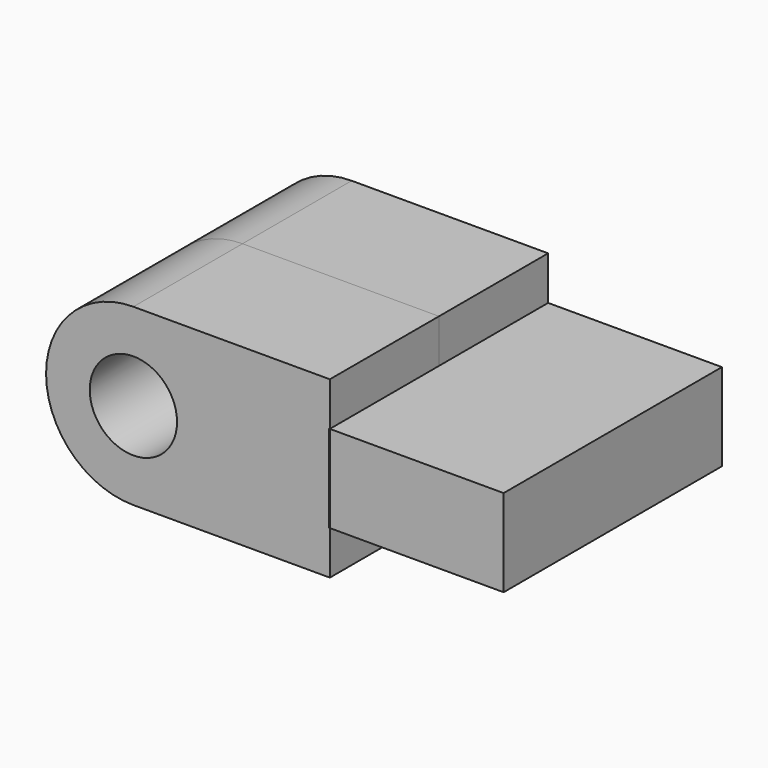
from build123d import *

# Parameters (mm, degrees)
F0_W     = 31.8502481282
F0_H     = 16
F1_DEPTH = 25
F0_R     = 8


with BuildPart() as f1:
    # F0 (on Front) → F1 (new body)
    with BuildSketch(Plane.XZ):
        with Locations((51.9251240641, 0)):
            Rectangle(F0_W, F0_H)
    extrude(amount=F1_DEPTH)

    # F3: F1 across plane


with BuildPart() as f1b:
    # F0 (on Front) → F1, piece 2 (new body)
    with BuildSketch(Plane.XZ):
        with BuildLine():
            Line((36, 16), (0, 16))
            ThreePointArc((0, 16), (-16, 0), (0, -16))
            Line((0, -16), (36, -16))
            Line((36, -16), (36, -8))
            Line((36, -8), (35.8502481282, -8))
            Line((35.8502481282, -8), (35.8502481282, 8))
            Line((35.8502481282, 8), (36, 8))
            Line((36, 8), (36, 16))
        make_face()
        Circle(F0_R, mode=Mode.SUBTRACT)
    extrude(amount=F1_DEPTH)


with BuildPart() as f2_1:
    # F2: instance of F1b
    add(f1b.part.mirror(Plane.XZ))


with BuildPart() as f1_1:
    add(f1.part)
    add(f1.part.mirror(Plane.XZ))


solid = Compound([f1b.part, f2_1.part, f1_1.part])
